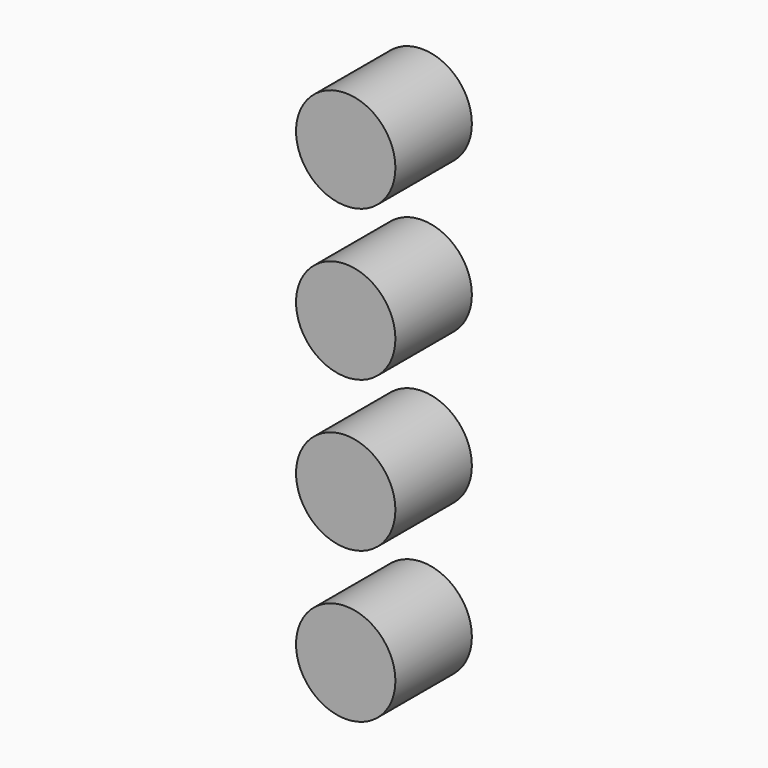
from build123d import *

# Parameters (mm, degrees)
F0_R     = 1.65
F1_DEPTH = 3.175


# Not quite as in the source:
# - a length typed as a fraction of an inch, garbled in the dataset ("3 / 203.2 mm" for 3/8 in), is restored


with BuildPart() as f1:
    # F0 (on Front) → F1 (new body)
    with BuildSketch(Plane.XZ):
        with Locations((0, 35)):
            Circle(F0_R)
    extrude(amount=F1_DEPTH)


with BuildPart() as f1b:
    # F0 (on Front) → F1, piece 2 (new body)
    with BuildSketch(Plane.XZ):
        with Locations((0, 30)):
            Circle(F0_R)
    extrude(amount=F1_DEPTH)


with BuildPart() as f1c:
    # F0 (on Front) → F1, piece 3 (new body)
    with BuildSketch(Plane.XZ):
        with Locations((0, 25)):
            Circle(F0_R)
    extrude(amount=F1_DEPTH)


with BuildPart() as f1d:
    # F0 (on Front) → F1, piece 4 (new body)
    with BuildSketch(Plane.XZ):
        with Locations((0, 20)):
            Circle(F0_R)
    extrude(amount=F1_DEPTH)


solid = Compound([f1.part, f1b.part, f1c.part, f1d.part])
